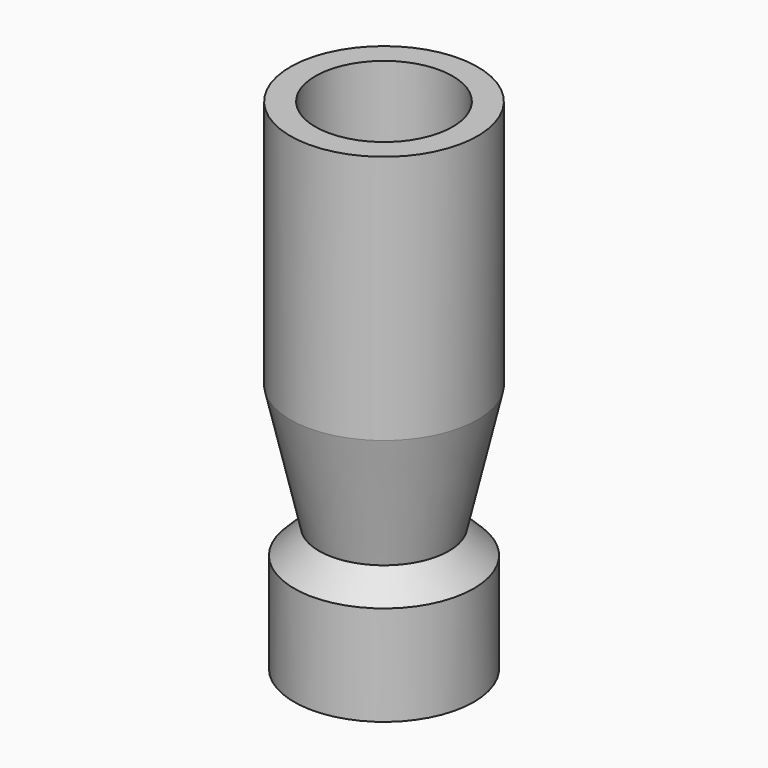
from build123d import *

# Parameters (mm, degrees)
F0_R     = 9.144
F0_R_2   = 6.604
F1_DEPTH = 12.7
F4_R     = 6.604
F4_R_2   = 4.064
F5_DEPTH = 2.54
F2_W     = 2.54
F2_H     = 25.4
F7_SIZE  = 2.53999


# Not quite as in the source:
# - a fillet or chamfer is up to 0.001 mm smaller than in the source, because OpenCascade refuses the exact size


with BuildPart() as f1:
    # F0 (on Top) → F1 (new body)
    with BuildSketch(Plane.XY):
        Circle(F0_R)
        Circle(F0_R_2, mode=Mode.SUBTRACT)
    extrude(amount=F1_DEPTH)

    # F4 (on offset) → F5 (join)
    with BuildSketch(Plane.XY.offset(12.7)):
        Circle(F4_R)
        Circle(F4_R_2, mode=Mode.SUBTRACT)
    extrude(amount=-F5_DEPTH)

    # F2 (on Right) → F6 (revolve)
    with BuildSketch(Plane.YZ):
        Polygon((-9.525, 25.4), (-6.604, 12.7), (-4.064, 12.7), (-6.985, 25.4), align=None)
        with Locations((-8.255, 38.1)):
            Rectangle(F2_W, F2_H)
    revolve(axis=Axis((0, 0, 0), (0, 0, 1)))

    # F7 (size 2.54 in the source; OpenCascade refuses exactly that, so slightly less here)
    f7_edges = [f1.edges().sort_by_distance(p)[0] for p in [
        (-9.144, 0, 12.7),
    ]]
    chamfer(f7_edges, length=F7_SIZE)


solid = f1.part
